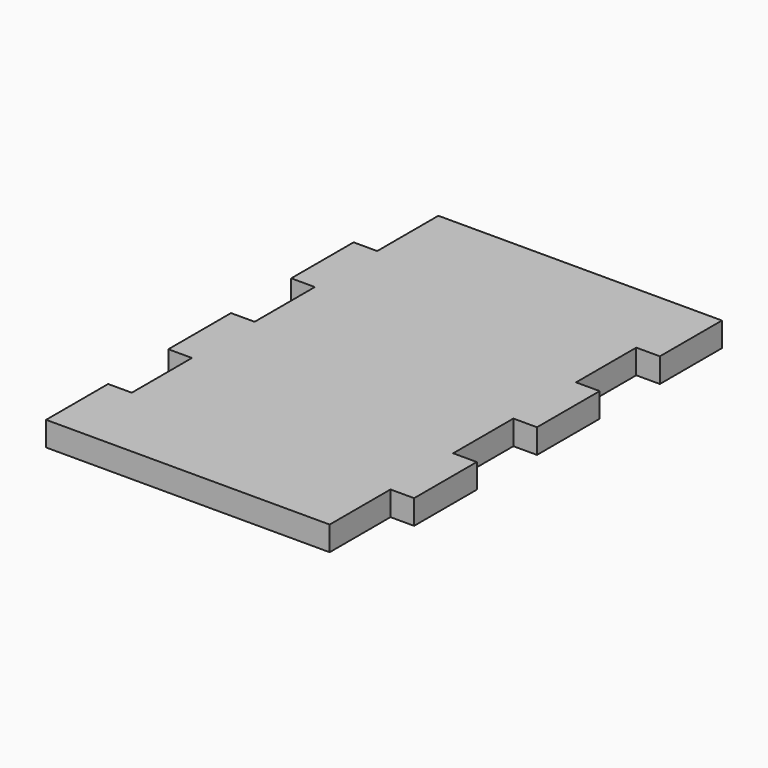
from build123d import *

# Parameters (mm, degrees)
F0_W     = 40
F0_H     = 60
F1_DEPTH = 3.175
F2_W     = 3.075
F2_H     = 9.9
F2_H_2   = 9.8
F2_H_3   = 9.95
F3_DEPTH = 25


# Not quite as in the source:
# - a length typed as a fraction of an inch, garbled in the dataset ("3 / 203.2 mm" for 3/8 in), is restored


with BuildPart() as f1:
    # F0 (on Top) → F1 (new body)
    with BuildSketch(Plane.XY):
        Rectangle(F0_W, F0_H)
    extrude(amount=F1_DEPTH)

    # F2 (on face) → F3 (cut)
    with BuildSketch(Plane.XY.offset(3.175)):
        with Locations((18.4625, -25.05)):
            Rectangle(F2_W, F2_H)
        with Locations((18.4625, -5)):
            Rectangle(F2_W, F2_H_2)
        with Locations((18.4625, 15)):
            Rectangle(F2_W, F2_H_2)
        with Locations((-18.4625, -15)):
            Rectangle(F2_W, F2_H_2)
        with Locations((-18.4625, 5)):
            Rectangle(F2_W, F2_H_2)
        with Locations((-18.4625, 25.025)):
            Rectangle(F2_W, F2_H_3)
    extrude(amount=-F3_DEPTH, mode=Mode.SUBTRACT)


solid = f1.part
